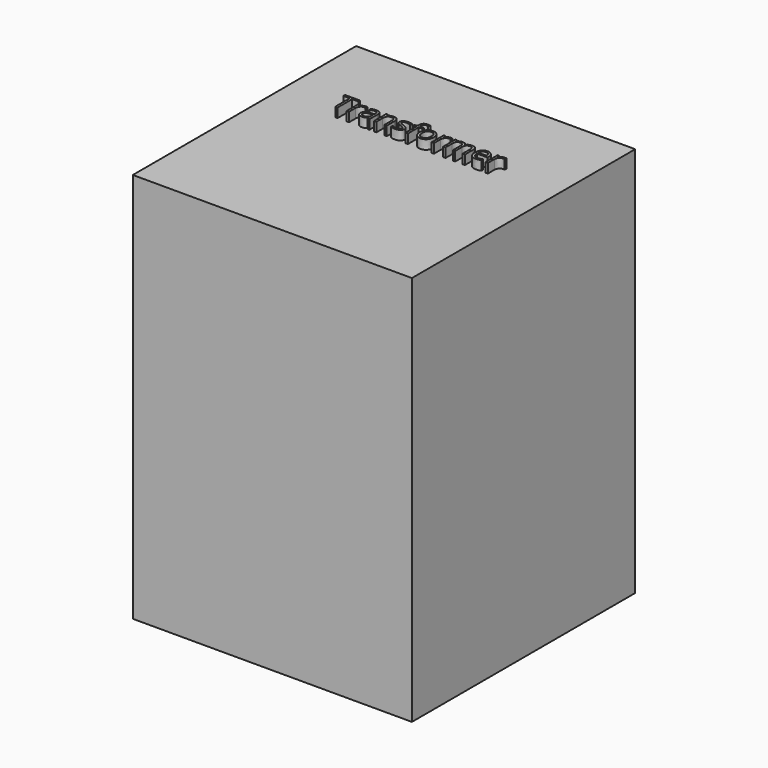
from build123d import *

# Parameters (mm, degrees)
F0_W         = 762
F0_H         = 762
F1_DEPTH     = 1066.8
F2_TEXT_SIZE = 77.3624514184
F3_DEPTH     = 25.4


# Not quite as in the source:
# - Text() gives the source's letters only with a copy of the font that has no kerning and outlines rounded to 1/6400 em; it was checked with that copy


with BuildPart() as f1:
    # F0 (on Top) → F1 (new body)
    with BuildSketch(Plane.XY):
        Rectangle(F0_W, F0_H)
    extrude(amount=F1_DEPTH)

    # F2 (on face) → F3 (join)
    with BuildSketch(Plane.XY.offset(1066.8)):
        with Locations((-228.6, 96.6990349787)):
            Text('Transformer', F2_TEXT_SIZE, font='Open Sans', text_align=(TextAlign.LEFT, TextAlign.BOTTOM))
    extrude(amount=F3_DEPTH)


solid = f1.part
